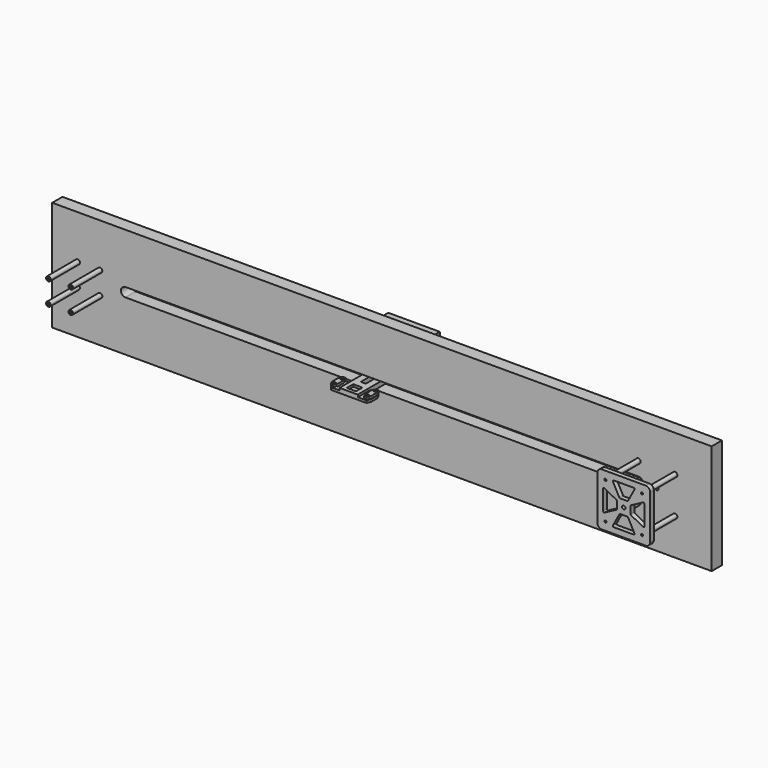
from build123d import *

# Parameters (mm, degrees)
F1_DEPTH       = 6
F2_W           = 8
F2_H           = 7.235
F3_DEPTH       = 6
F6_DEPTH       = 7.62
F8_DEPTH       = 7.62
F9_W           = 8
F9_H           = 3.175
F10_DEPTH      = 7.62
F10_DEPTH_BACK = 13.62
F12_DEPTH      = 7.236
F14_DEPTH      = 19.05
F14_DEPTH_BACK = 3.81
F17_DEPTH      = 7.236
F18_W          = 6.3396086097
F18_H          = 5.2124624596
F18_W_2        = 12.7207827806
F18_H_2        = 4.8503658202
F18_W_3        = 6.3603913903
F19_DEPTH      = 3.175
F19_DEPTH_BACK = 3.175
F20_R          = 1.905
F21_DEPTH      = 6.351
F22_W          = 7.0159770548
F22_H          = 37.1222775429
F23_DEPTH      = 6.351
F26_DEPTH      = 19.05
F27_W          = 15.0859798895
F27_H          = 38.1
F28_DEPTH      = 6.35
F29_TEXT_SIZE  = 21.1979624712
F30_DEPTH      = 3.175
F32_W          = 914.4
F32_H          = 152.4
F32_R          = 1.24968
F32_R_2        = 2.38125
F33_DEPTH      = 17.78
F34_R          = 3.175
F34_R_2        = 1.4605
F35_DEPTH      = 50.8
F36_R          = 1.4605
F36_R_2        = 2.38125
F37_DEPTH      = 6.35


# Not quite as in the source:
# - Text() gives the source's letters only with a copy of the font that has no kerning and outlines rounded to 1/6400 em; it was checked with that copy


with BuildPart() as f1:
    # F0 (on Front) → F1 (new body)
    with BuildSketch(Plane.XZ):
        with BuildLine():
            Line((0.2044851016, 0), (0, 0))
            Line((0, 0), (0, -0.76))
            Line((0, -0.76), (16, -0.76))
            Line((16, -0.76), (16, 0))
            Line((16, 0), (15.7955148984, 0))
            ThreePointArc((15.7955148984, 0), (15.7149199572, 0.0234912831), (15.6595687304, 0.0866072607))
            Line((15.6595687304, 0.0866072607), (15.3859461681, 0.6733927393))
            ThreePointArc((15.3859461681, 0.6733927393), (15.3305949413, 0.7365087169), (15.25, 0.76))
            Line((15.25, 0.76), (14.75, 0.76))
            ThreePointArc((14.75, 0.76), (14.6694050587, 0.7365087169), (14.6140538319, 0.6733927393))
            Line((14.6140538319, 0.6733927393), (14.3404312696, 0.0866072607))
            ThreePointArc((14.3404312696, 0.0866072607), (14.2850800428, 0.0234912831), (14.2044851016, 0))
            Line((14.2044851016, 0), (14, 0))
            Line((14, 0), (13.7955148984, 0))
            ThreePointArc((13.7955148984, 0), (13.7149199572, 0.0234912831), (13.6595687304, 0.0866072607))
            Line((13.6595687304, 0.0866072607), (13.3859461681, 0.6733927393))
            ThreePointArc((13.3859461681, 0.6733927393), (13.3305949413, 0.7365087169), (13.25, 0.76))
            Line((13.25, 0.76), (12.75, 0.76))
            ThreePointArc((12.75, 0.76), (12.6694050587, 0.7365087169), (12.6140538319, 0.6733927393))
            Line((12.6140538319, 0.6733927393), (12.3404312696, 0.0866072607))
            ThreePointArc((12.3404312696, 0.0866072607), (12.2850800428, 0.0234912831), (12.2044851016, 0))
            Line((12.2044851016, 0), (12, 0))
            Line((12, 0), (11.7955148984, 0))
            ThreePointArc((11.7955148984, 0), (11.7149199572, 0.0234912831), (11.6595687304, 0.0866072607))
            Line((11.6595687304, 0.0866072607), (11.3859461681, 0.6733927393))
            ThreePointArc((11.3859461681, 0.6733927393), (11.3305949413, 0.7365087169), (11.25, 0.76))
            Line((11.25, 0.76), (10.75, 0.76))
            ThreePointArc((10.75, 0.76), (10.6694050587, 0.7365087169), (10.6140538319, 0.6733927393))
            Line((10.6140538319, 0.6733927393), (10.3404312696, 0.0866072607))
            ThreePointArc((10.3404312696, 0.0866072607), (10.2850800428, 0.0234912831), (10.2044851016, 0))
            Line((10.2044851016, 0), (10, 0))
            Line((10, 0), (9.7955148984, 0))
            ThreePointArc((9.7955148984, 0), (9.7149199572, 0.0234912831), (9.6595687304, 0.0866072607))
            Line((9.6595687304, 0.0866072607), (9.3859461681, 0.6733927393))
            ThreePointArc((9.3859461681, 0.6733927393), (9.3305949413, 0.7365087169), (9.25, 0.76))
            Line((9.25, 0.76), (8.75, 0.76))
            ThreePointArc((8.75, 0.76), (8.6694050587, 0.7365087169), (8.6140538319, 0.6733927393))
            Line((8.6140538319, 0.6733927393), (8.3404312696, 0.0866072607))
            ThreePointArc((8.3404312696, 0.0866072607), (8.2850800428, 0.0234912831), (8.2044851016, 0))
            Line((8.2044851016, 0), (8, 0))
            Line((8, 0), (7.7955148984, 0))
            ThreePointArc((7.7955148984, 0), (7.7149199572, 0.0234912831), (7.6595687304, 0.0866072607))
            Line((7.6595687304, 0.0866072607), (7.3859461681, 0.6733927393))
            ThreePointArc((7.3859461681, 0.6733927393), (7.3305949413, 0.7365087169), (7.25, 0.76))
            Line((7.25, 0.76), (6.75, 0.76))
            ThreePointArc((6.75, 0.76), (6.6694050587, 0.7365087169), (6.6140538319, 0.6733927393))
            Line((6.6140538319, 0.6733927393), (6.3404312696, 0.0866072607))
            ThreePointArc((6.3404312696, 0.0866072607), (6.2850800428, 0.0234912831), (6.2044851016, 0))
            Line((6.2044851016, 0), (6, 0))
            Line((6, 0), (5.7955148984, 0))
            ThreePointArc((5.7955148984, 0), (5.7149199572, 0.0234912831), (5.6595687304, 0.0866072607))
            Line((5.6595687304, 0.0866072607), (5.3859461681, 0.6733927393))
            ThreePointArc((5.3859461681, 0.6733927393), (5.3305949413, 0.7365087169), (5.25, 0.76))
            Line((5.25, 0.76), (4.75, 0.76))
            ThreePointArc((4.75, 0.76), (4.6694050587, 0.7365087169), (4.6140538319, 0.6733927393))
            Line((4.6140538319, 0.6733927393), (4.3404312696, 0.0866072607))
            ThreePointArc((4.3404312696, 0.0866072607), (4.2850800428, 0.0234912831), (4.2044851016, 0))
            Line((4.2044851016, 0), (4, 0))
            Line((4, 0), (3.7955148984, 0))
            ThreePointArc((3.7955148984, 0), (3.7149199572, 0.0234912831), (3.6595687304, 0.0866072607))
            Line((3.6595687304, 0.0866072607), (3.3859461681, 0.6733927393))
            ThreePointArc((3.3859461681, 0.6733927393), (3.3305949413, 0.7365087169), (3.25, 0.76))
            Line((3.25, 0.76), (2.75, 0.76))
            ThreePointArc((2.75, 0.76), (2.6694050587, 0.7365087169), (2.6140538319, 0.6733927393))
            Line((2.6140538319, 0.6733927393), (2.3404312696, 0.0866072607))
            ThreePointArc((2.3404312696, 0.0866072607), (2.2850800428, 0.0234912831), (2.2044851016, 0))
            Line((2.2044851016, 0), (2, 0))
            Line((2, 0), (1.7955148984, 0))
            ThreePointArc((1.7955148984, 0), (1.7149199572, 0.0234912831), (1.6595687304, 0.0866072607))
            Line((1.6595687304, 0.0866072607), (1.3859461681, 0.6733927393))
            ThreePointArc((1.3859461681, 0.6733927393), (1.3305949413, 0.7365087169), (1.25, 0.76))
            Line((1.25, 0.76), (0.75, 0.76))
            ThreePointArc((0.75, 0.76), (0.6694050587, 0.7365087169), (0.6140538319, 0.6733927393))
            Line((0.6140538319, 0.6733927393), (0.3404312696, 0.0866072607))
            ThreePointArc((0.3404312696, 0.0866072607), (0.2850800428, 0.0234912831), (0.2044851016, 0))
        make_face()
    extrude(amount=F1_DEPTH)


with BuildPart() as f3:
    # F2 (on face) → F3 (new body)
    with BuildSketch(Plane.XZ.offset(6)):
        with Locations((4, -0.3175)):
            Rectangle(F2_W, F2_H)
    extrude(amount=-F3_DEPTH)

    # F4: cut F1
    add(f1.part, mode=Mode.SUBTRACT)

    # F5 (on face) → F6 (join)
    with BuildSketch(Plane(origin=(0, 0, 0), x_dir=(-1, 0, 0), z_dir=(0, 1, 0))):
        with BuildLine():
            Line((0, 0), (0, 3.3))
            Line((0, 3.3), (-8, 3.3))
            Line((-8, 3.3), (-8, 0))
            Line((-8, 0), (-7.7955148984, 0))
            ThreePointArc((-7.7955148984, 0), (-7.7149199572, 0.0234912831), (-7.6595687304, 0.0866072607))
            Line((-7.6595687304, 0.0866072607), (-7.3859461681, 0.6733927393))
            ThreePointArc((-7.3859461681, 0.6733927393), (-7.3305949413, 0.7365087169), (-7.25, 0.76))
            Line((-7.25, 0.76), (-6.75, 0.76))
            ThreePointArc((-6.75, 0.76), (-6.6694050587, 0.7365087169), (-6.6140538319, 0.6733927393))
            Line((-6.6140538319, 0.6733927393), (-6.3404312696, 0.0866072607))
            ThreePointArc((-6.3404312696, 0.0866072607), (-6.2850800428, 0.0234912831), (-6.2044851016, 0))
            Line((-6.2044851016, 0), (-5.7955148984, 0))
            ThreePointArc((-5.7955148984, 0), (-5.7149199572, 0.0234912831), (-5.6595687304, 0.0866072607))
            Line((-5.6595687304, 0.0866072607), (-5.3859461681, 0.6733927393))
            ThreePointArc((-5.3859461681, 0.6733927393), (-5.3305949413, 0.7365087169), (-5.25, 0.76))
            Line((-5.25, 0.76), (-4.75, 0.76))
            ThreePointArc((-4.75, 0.76), (-4.6694050587, 0.7365087169), (-4.6140538319, 0.6733927393))
            Line((-4.6140538319, 0.6733927393), (-4.3404312696, 0.0866072607))
            ThreePointArc((-4.3404312696, 0.0866072607), (-4.2850800428, 0.0234912831), (-4.2044851016, 0))
            Line((-4.2044851016, 0), (-3.7955148984, 0))
            ThreePointArc((-3.7955148984, 0), (-3.7149199572, 0.0234912831), (-3.6595687304, 0.0866072607))
            Line((-3.6595687304, 0.0866072607), (-3.3859461681, 0.6733927393))
            ThreePointArc((-3.3859461681, 0.6733927393), (-3.3305949413, 0.7365087169), (-3.25, 0.76))
            Line((-3.25, 0.76), (-2.75, 0.76))
            ThreePointArc((-2.75, 0.76), (-2.6694050587, 0.7365087169), (-2.6140538319, 0.6733927393))
            Line((-2.6140538319, 0.6733927393), (-2.3404312696, 0.0866072607))
            ThreePointArc((-2.3404312696, 0.0866072607), (-2.2850800428, 0.0234912831), (-2.2044851016, 0))
            Line((-2.2044851016, 0), (-1.7955148984, 0))
            ThreePointArc((-1.7955148984, 0), (-1.7149199572, 0.0234912831), (-1.6595687304, 0.0866072607))
            Line((-1.6595687304, 0.0866072607), (-1.3859461681, 0.6733927393))
            ThreePointArc((-1.3859461681, 0.6733927393), (-1.3305949413, 0.7365087169), (-1.25, 0.76))
            Line((-1.25, 0.76), (-0.75, 0.76))
            ThreePointArc((-0.75, 0.76), (-0.6694050587, 0.7365087169), (-0.6140538319, 0.6733927393))
            Line((-0.6140538319, 0.6733927393), (-0.3404312696, 0.0866072607))
            ThreePointArc((-0.3404312696, 0.0866072607), (-0.2850800428, 0.0234912831), (-0.2044851016, 0))
            Line((-0.2044851016, 0), (0, 0))
        make_face()
    extrude(amount=F6_DEPTH)

    # F7 (on face) → F8 (join)
    with BuildSketch(Plane.XZ.offset(6)):
        with BuildLine():
            Line((8, 0), (8, 3.3))
            Line((8, 3.3), (0, 3.3))
            Line((0, 3.3), (0, 0))
            Line((0, 0), (0.2044851016, 0))
            ThreePointArc((0.2044851016, 0), (0.2850800428, 0.0234912831), (0.3404312696, 0.0866072607))
            Line((0.3404312696, 0.0866072607), (0.6140538319, 0.6733927393))
            ThreePointArc((0.6140538319, 0.6733927393), (0.6694050587, 0.7365087169), (0.75, 0.76))
            Line((0.75, 0.76), (1.25, 0.76))
            ThreePointArc((1.25, 0.76), (1.3305949413, 0.7365087169), (1.3859461681, 0.6733927393))
            Line((1.3859461681, 0.6733927393), (1.6595687304, 0.0866072607))
            ThreePointArc((1.6595687304, 0.0866072607), (1.7149199572, 0.0234912831), (1.7955148984, 0))
            Line((1.7955148984, 0), (2.2044851016, 0))
            ThreePointArc((2.2044851016, 0), (2.2850800428, 0.0234912831), (2.3404312696, 0.0866072607))
            Line((2.3404312696, 0.0866072607), (2.6140538319, 0.6733927393))
            ThreePointArc((2.6140538319, 0.6733927393), (2.6694050587, 0.7365087169), (2.75, 0.76))
            Line((2.75, 0.76), (3.25, 0.76))
            ThreePointArc((3.25, 0.76), (3.3305949413, 0.7365087169), (3.3859461681, 0.6733927393))
            Line((3.3859461681, 0.6733927393), (3.6595687304, 0.0866072607))
            ThreePointArc((3.6595687304, 0.0866072607), (3.7149199572, 0.0234912831), (3.7955148984, 0))
            Line((3.7955148984, 0), (4.2044851016, 0))
            ThreePointArc((4.2044851016, 0), (4.2850800428, 0.0234912831), (4.3404312696, 0.0866072607))
            Line((4.3404312696, 0.0866072607), (4.6140538319, 0.6733927393))
            ThreePointArc((4.6140538319, 0.6733927393), (4.6694050587, 0.7365087169), (4.75, 0.76))
            Line((4.75, 0.76), (5.25, 0.76))
            ThreePointArc((5.25, 0.76), (5.3305949413, 0.7365087169), (5.3859461681, 0.6733927393))
            Line((5.3859461681, 0.6733927393), (5.6595687304, 0.0866072607))
            ThreePointArc((5.6595687304, 0.0866072607), (5.7149199572, 0.0234912831), (5.7955148984, 0))
            Line((5.7955148984, 0), (6.2044851016, 0))
            ThreePointArc((6.2044851016, 0), (6.2850800428, 0.0234912831), (6.3404312696, 0.0866072607))
            Line((6.3404312696, 0.0866072607), (6.6140538319, 0.6733927393))
            ThreePointArc((6.6140538319, 0.6733927393), (6.6694050587, 0.7365087169), (6.75, 0.76))
            Line((6.75, 0.76), (7.25, 0.76))
            ThreePointArc((7.25, 0.76), (7.3305949413, 0.7365087169), (7.3859461681, 0.6733927393))
            Line((7.3859461681, 0.6733927393), (7.6595687304, 0.0866072607))
            ThreePointArc((7.6595687304, 0.0866072607), (7.7149199572, 0.0234912831), (7.7955148984, 0))
            Line((7.7955148984, 0), (8, 0))
        make_face()
    extrude(amount=F8_DEPTH)

    # F9 (on face) → F10 (join, two sides)
    with BuildSketch(Plane(origin=(0, 0, 0), x_dir=(-1, 0, 0), z_dir=(0, 1, 0))) as f10_sk:
        with Locations((-4, -2.3475)):
            Rectangle(F9_W, F9_H)
    extrude(amount=F10_DEPTH)
    extrude(f10_sk.sketch, amount=-F10_DEPTH_BACK)

    # F11 (on face) → F12 (cut, through all)
    with BuildSketch(Plane.XY.offset(3.3)):
        Polygon((8, -13.62), (8, -8.54), (5.5875, -13.62), align=None)
        Polygon((0, -13.62), (2.4125, -13.62), (0, -8.54), align=None)
        Polygon((5.5875, 7.62), (8, 2.54), (8, 7.62), align=None)
        Polygon((0, 7.62), (0, 2.54), (2.4125, 7.62), align=None)
    extrude(amount=-F12_DEPTH, mode=Mode.SUBTRACT)

    # F13 (on face) → F14 (join, two sides)
    with BuildSketch(Plane(origin=(0, 0, 0), x_dir=(0, -1, 0), z_dir=(-1, 0, 0))) as f14_sk:
        Polygon((-7.62, -0.76), (-7.62, -3.935), (-2.54, -3.935), (8.54, -3.935), (13.62, -3.935), (13.62, -0.76), (8.54, -0.76), (-2.54, -0.76), align=None)
    extrude(amount=F14_DEPTH)
    extrude(f14_sk.sketch, amount=-F14_DEPTH_BACK)

    # F15: F3 across face


with BuildPart() as f3_1:
    add(f3.part)
    add(f3.part.mirror(Plane(origin=(-19.05, -3, -2.3475), x_dir=(0, -1, 0), z_dir=(-1, 0, 0))))

    # F16 (on face) → F17 (cut, through all)
    with BuildSketch(Plane.XY.offset(3.3)):
        with BuildLine():
            Line((4.064, 3.35), (2.413, 3.35))
            ThreePointArc((2.413, 3.35), (2.8965667043, 2.1825667043), (4.064, 1.699))
            Line((4.064, 1.699), (4.064, 3.35))
        make_face()
        with BuildLine():
            ThreePointArc((5.715, 3.35), (4.064, 5.001), (2.413, 3.35))
            Line((2.413, 3.35), (4.064, 3.35))
            Line((4.064, 3.35), (4.064, 1.699))
            ThreePointArc((4.064, 1.699), (5.2314332957, 2.1825667043), (5.715, 3.35))
        make_face()
        with BuildLine():
            Line((4.064, -9.35), (4.064, -7.699))
            ThreePointArc((4.064, -7.699), (2.8965667043, -8.1825667043), (2.413, -9.35))
            Line((2.413, -9.35), (4.064, -9.35))
        make_face()
        with BuildLine():
            ThreePointArc((5.715, -9.35), (5.2314332957, -8.1825667043), (4.064, -7.699))
            Line((4.064, -7.699), (4.064, -9.35))
            Line((4.064, -9.35), (2.413, -9.35))
            ThreePointArc((2.413, -9.35), (4.064, -11.001), (5.715, -9.35))
        make_face()
        with BuildLine():
            Line((-42.164, 3.35), (-40.513, 3.35))
            ThreePointArc((-40.513, 3.35), (-43.3314332957, 4.5174332957), (-42.164, 1.699))
            Line((-42.164, 1.699), (-42.164, 3.35))
        make_face()
        with BuildLine():
            ThreePointArc((-42.164, 1.699), (-40.9965667043, 2.1825667043), (-40.513, 3.35))
            Line((-40.513, 3.35), (-42.164, 3.35))
            Line((-42.164, 3.35), (-42.164, 1.699))
        make_face()
        with BuildLine():
            Line((-42.164, -9.35), (-42.164, -7.699))
            ThreePointArc((-42.164, -7.699), (-43.3314332957, -10.5174332957), (-40.513, -9.35))
            Line((-40.513, -9.35), (-42.164, -9.35))
        make_face()
        with BuildLine():
            ThreePointArc((-40.513, -9.35), (-40.9965667043, -8.1825667043), (-42.164, -7.699))
            Line((-42.164, -7.699), (-42.164, -9.35))
            Line((-42.164, -9.35), (-40.513, -9.35))
        make_face()
    extrude(amount=-F17_DEPTH, mode=Mode.SUBTRACT)

    # F18 (on face) → F19 (join, two sides)
    with BuildSketch(Plane.XY.offset(-0.76)) as f19_sk:
        Polygon((-12.6896086097, -8.7696341798), (-6.35, -8.7696341798), (-6.35, 2.4075375404), (-12.6896086097, 2.4075375404), (-12.6896086097, -3), align=None)
        with Locations((-9.5198043048, 5.0137687702)):
            Rectangle(F18_W, F18_H)
        with Locations((-19.05, 5.0137687702)):
            Rectangle(F18_W_2, F18_H)
        with Locations((-28.5801956952, 5.0137687702)):
            Rectangle(F18_W, F18_H)
        Polygon((-31.75, -8.7696341798), (-25.4103913903, -8.7696341798), (-25.4103913903, -3), (-25.4103913903, 2.4075375404), (-31.75, 2.4075375404), align=None)
        with Locations((-28.5801956952, -11.1948170899)):
            Rectangle(F18_W, F18_H_2)
        with Locations((-15.8698043048, -11.1948170899)):
            Rectangle(F18_W_3, F18_H_2)
        with Locations((-22.2301956952, -11.1948170899)):
            Rectangle(F18_W_3, F18_H_2)
        with Locations((-9.5198043048, -11.1948170899)):
            Rectangle(F18_W, F18_H_2)
        with BuildLine():
            Line((-12.6896086097, 7.62), (-6.35, 7.62))
            Line((-6.35, 7.62), (-6.35, 71.12))
            ThreePointArc((-6.35, 71.12), (-19.05, 83.82), (-31.75, 71.12))
            Line((-31.75, 71.12), (-31.75, 7.62))
            Line((-31.75, 7.62), (-25.4103913903, 7.62))
            Line((-25.4103913903, 7.62), (-12.6896086097, 7.62))
        make_face()
    extrude(amount=F19_DEPTH)
    extrude(f19_sk.sketch, amount=-F19_DEPTH_BACK)

    # F20 (on face) → F21 (cut, through all)
    with BuildSketch(Plane.XY.offset(2.415)):
        with BuildLine():
            ThreePointArc((-16.1925, 72.2575375404), (-14.2875, 70.3525375404), (-12.3825, 72.2575375404))
            ThreePointArc((-12.3825, 72.2575375404), (-14.2875, 74.1625375404), (-16.1925, 72.2575375404))
        make_face()
        with Locations((-23.8125, 72.2575375404)):
            Circle(F20_R)
    extrude(amount=-F21_DEPTH, mode=Mode.SUBTRACT)

    # F22 (on face) → F23 (cut, through all)
    with BuildSketch(Plane.XY.offset(2.415)):
        with Locations((-19.022686407, 30.2847372368)):
            Rectangle(F22_W, F22_H)
    extrude(amount=-F23_DEPTH, mode=Mode.SUBTRACT)


with BuildPart() as f26:
    # F25 (on 3pt) → F26 (new body, symmetric)
    with BuildSketch(Plane.XZ.offset(-71.12)):
        Polygon((-19.05, 8.765), (31.75, 8.765), (44.45, 34.165), (-19.05, 34.165), align=None)
        Polygon((-69.85, 8.765), (-19.05, 8.765), (-19.05, 34.165), (-82.55, 34.165), align=None)
    extrude(amount=F26_DEPTH, both=True)

    # F27 (on face) → F28 (join)
    with BuildSketch(Plane.XY.offset(34.165)):
        with Locations((24.2070100553, 71.12)):
            Rectangle(F27_W, F27_H)
        Polygon((16.6640201105, 42.545), (16.6640201105, 52.07), (4.7593467403, 52.07), align=None)
        Polygon((4.7593467403, 52.07), (16.6640201105, 52.07), (16.6640201105, 90.17), (-42.8593467403, 90.17), align=None)
        Polygon((16.6640201105, 42.545), (4.7593467403, 52.07), (-54.7640201105, 52.07), (-54.7640201105, 42.545), align=None)
        Polygon((-54.7640201105, 52.07), (4.7593467403, 52.07), (-42.8593467403, 90.17), (-54.7640201105, 90.17), align=None)
        Polygon((-42.8593467403, 90.17), (16.6640201105, 90.17), (16.6640201105, 99.695), (-54.7640201105, 99.695), align=None)
        with Locations((-62.3070100553, 71.12)):
            Rectangle(F27_W, F27_H)
        Polygon((-54.7640201105, 90.17), (-42.8593467403, 90.17), (-54.7640201105, 99.695), align=None)
    extrude(amount=F28_DEPTH)

    # F29 (on face) → F30 (cut)
    with BuildSketch(Plane.XY.offset(40.515)):
        with Locations((-30.2830450237, 47.0722429454)):
            Text('X', F29_TEXT_SIZE, font='Open Sans', text_align=(TextAlign.LEFT, TextAlign.BOTTOM))
    extrude(amount=-F30_DEPTH, mode=Mode.SUBTRACT)


with BuildPart() as f33:
    # F32 (on offset) → F33 (new body)
    with BuildSketch(Plane.XZ.offset(-20.32)):
        Rectangle(F32_W, F32_H)
        with Locations((-421.90035, -15.50035)):
            Circle(F32_R, mode=Mode.SUBTRACT)
        with Locations((-390.89965, -15.50035)):
            Circle(F32_R, mode=Mode.SUBTRACT)
        with Locations((355.6, -25.4)):
            Circle(F32_R, mode=Mode.SUBTRACT)
        with Locations((406.4, -25.4)):
            Circle(F32_R, mode=Mode.SUBTRACT)
        with Locations((-421.90035, 15.50035)):
            Circle(F32_R, mode=Mode.SUBTRACT)
        with Locations((-390.89965, 15.50035)):
            Circle(F32_R, mode=Mode.SUBTRACT)
        with BuildLine():
            Line((-355.6, 6.35), (355.6, 6.35))
            ThreePointArc((355.6, 6.35), (361.95, 0), (355.6, -6.35))
            Line((355.6, -6.35), (-355.6, -6.35))
            ThreePointArc((-355.6, -6.35), (-361.95, 0), (-355.6, 6.35))
        make_face(mode=Mode.SUBTRACT)
        with Locations((381, 0)):
            Circle(F32_R_2, mode=Mode.SUBTRACT)
        with Locations((355.6, 25.4)):
            Circle(F32_R, mode=Mode.SUBTRACT)
        with Locations((406.4, 25.4)):
            Circle(F32_R, mode=Mode.SUBTRACT)
    extrude(amount=-F33_DEPTH)


with BuildPart() as f35:
    # F34 (on face) → F35 (new body)
    with BuildSketch(Plane.XZ.offset(-20.32)):
        with Locations((-421.90035, 15.50035)):
            Circle(F34_R)
        with Locations((-421.90035, 15.50035)):
            Circle(F34_R_2, mode=Mode.SUBTRACT)
    extrude(amount=F35_DEPTH)


with BuildPart() as f35b:
    # F34 (on face) → F35, piece 2 (new body)
    with BuildSketch(Plane.XZ.offset(-20.32)):
        with Locations((-390.89965, 15.50035)):
            Circle(F34_R)
        with Locations((-390.89965, 15.50035)):
            Circle(F34_R_2, mode=Mode.SUBTRACT)
    extrude(amount=F35_DEPTH)


with BuildPart() as f35c:
    # F34 (on face) → F35, piece 3 (new body)
    with BuildSketch(Plane.XZ.offset(-20.32)):
        with Locations((-390.89965, -15.50035)):
            Circle(F34_R)
        with Locations((-390.89965, -15.50035)):
            Circle(F34_R_2, mode=Mode.SUBTRACT)
    extrude(amount=F35_DEPTH)


with BuildPart() as f35d:
    # F34 (on face) → F35, piece 4 (new body)
    with BuildSketch(Plane.XZ.offset(-20.32)):
        with Locations((-421.90035, -15.50035)):
            Circle(F34_R)
        with Locations((-421.90035, -15.50035)):
            Circle(F34_R_2, mode=Mode.SUBTRACT)
    extrude(amount=F35_DEPTH)


with BuildPart() as f35e:
    # F34 (on face) → F35, piece 5 (new body)
    with BuildSketch(Plane.XZ.offset(-20.32)):
        with Locations((406.4, 25.4)):
            Circle(F34_R)
        with Locations((406.4, 25.4)):
            Circle(F34_R_2, mode=Mode.SUBTRACT)
    extrude(amount=F35_DEPTH)


with BuildPart() as f35f:
    # F34 (on face) → F35, piece 6 (new body)
    with BuildSketch(Plane.XZ.offset(-20.32)):
        with Locations((355.6, 25.4)):
            Circle(F34_R)
        with Locations((355.6, 25.4)):
            Circle(F34_R_2, mode=Mode.SUBTRACT)
    extrude(amount=F35_DEPTH)


with BuildPart() as f35g:
    # F34 (on face) → F35, piece 7 (new body)
    with BuildSketch(Plane.XZ.offset(-20.32)):
        with Locations((355.6, -25.4)):
            Circle(F34_R)
        with Locations((355.6, -25.4)):
            Circle(F34_R_2, mode=Mode.SUBTRACT)
    extrude(amount=F35_DEPTH)


with BuildPart() as f35h:
    # F34 (on face) → F35, piece 8 (new body)
    with BuildSketch(Plane.XZ.offset(-20.32)):
        with Locations((406.4, -25.4)):
            Circle(F34_R)
        with Locations((406.4, -25.4)):
            Circle(F34_R_2, mode=Mode.SUBTRACT)
    extrude(amount=F35_DEPTH)


with BuildPart() as f37:
    # F36 (on face) → F37 (new body)
    with BuildSketch(Plane.XZ.offset(30.48)):
        with BuildLine():
            ThreePointArc((417.6395, 30.2895), (415.7796280605, 34.7796280605), (411.2895, 36.6395))
            Line((411.2895, 36.6395), (350.7105, 36.6395))
            ThreePointArc((350.7105, 36.6395), (346.2203719395, 34.7796280605), (344.3605, 30.2895))
            Line((344.3605, 30.2895), (344.3605, -30.2895))
            ThreePointArc((344.3605, -30.2895), (346.2203719395, -34.7796280605), (350.7105, -36.6395))
            Line((350.7105, -36.6395), (411.2895, -36.6395))
            ThreePointArc((411.2895, -36.6395), (415.7796280605, -34.7796280605), (417.6395, -30.2895))
            Line((417.6395, -30.2895), (417.6395, 30.2895))
        make_face()
        with Locations((355.6, -25.4)):
            Circle(F36_R, mode=Mode.SUBTRACT)
        with BuildLine():
            Line((394.7583333333, -28.575), (367.2416666667, -28.575))
            ThreePointArc((367.2416666667, -28.575), (366.152650651, -27.9584096094), (366.1210784314, -26.7073529412))
            Line((366.1210784314, -26.7073529412), (374.9264117647, -10.1973529412))
            ThreePointArc((374.9264117647, -10.1973529412), (375.3935903906, -9.7059839843), (376.047, -9.525))
            Line((376.047, -9.525), (385.953, -9.525))
            ThreePointArc((385.953, -9.525), (386.6064096094, -9.7059839843), (387.0735882353, -10.1973529412))
            Line((387.0735882353, -10.1973529412), (395.8789215686, -26.7073529412))
            ThreePointArc((395.8789215686, -26.7073529412), (395.847349349, -27.9584096094), (394.7583333333, -28.575))
        make_face(mode=Mode.SUBTRACT)
        with Locations((406.4, -25.4)):
            Circle(F36_R, mode=Mode.SUBTRACT)
        with BuildLine():
            Line((352.425, -13.7583333333), (352.425, 13.7583333333))
            ThreePointArc((352.425, 13.7583333333), (353.0415903906, 14.847349349), (354.2926470588, 14.8789215686))
            Line((354.2926470588, 14.8789215686), (370.8026470588, 6.0735882353))
            ThreePointArc((370.8026470588, 6.0735882353), (371.2940160156, 5.6064096094), (371.475, 4.953))
            Line((371.475, 4.953), (371.475, -4.953))
            ThreePointArc((371.475, -4.953), (371.2940160156, -5.6064096094), (370.8026470588, -6.0735882353))
            Line((370.8026470588, -6.0735882353), (354.2926470588, -14.8789215686))
            ThreePointArc((354.2926470588, -14.8789215686), (353.0415903906, -14.847349349), (352.425, -13.7583333333))
        make_face(mode=Mode.SUBTRACT)
        with Locations((381, 0)):
            Circle(F36_R_2, mode=Mode.SUBTRACT)
        with Locations((355.6, 25.4)):
            Circle(F36_R, mode=Mode.SUBTRACT)
        with BuildLine():
            ThreePointArc((366.1210784314, 26.7073529412), (366.152650651, 27.9584096094), (367.2416666667, 28.575))
            Line((367.2416666667, 28.575), (394.7583333333, 28.575))
            ThreePointArc((394.7583333333, 28.575), (395.847349349, 27.9584096094), (395.8789215686, 26.7073529412))
            Line((395.8789215686, 26.7073529412), (387.0735882353, 10.1973529412))
            ThreePointArc((387.0735882353, 10.1973529412), (386.6064096094, 9.7059839843), (385.953, 9.525))
            Line((385.953, 9.525), (376.047, 9.525))
            ThreePointArc((376.047, 9.525), (375.3935903906, 9.7059839843), (374.9264117647, 10.1973529412))
            Line((374.9264117647, 10.1973529412), (366.1210784314, 26.7073529412))
        make_face(mode=Mode.SUBTRACT)
        with BuildLine():
            Line((391.1973529412, 6.0735882353), (407.7073529412, 14.8789215686))
            ThreePointArc((407.7073529412, 14.8789215686), (408.9584096094, 14.847349349), (409.575, 13.7583333333))
            Line((409.575, 13.7583333333), (409.575, -13.7583333333))
            ThreePointArc((409.575, -13.7583333333), (408.9584096094, -14.847349349), (407.7073529412, -14.8789215686))
            Line((407.7073529412, -14.8789215686), (391.1973529412, -6.0735882353))
            ThreePointArc((391.1973529412, -6.0735882353), (390.7059839843, -5.6064096094), (390.525, -4.953))
            Line((390.525, -4.953), (390.525, 4.953))
            ThreePointArc((390.525, 4.953), (390.7059839843, 5.6064096094), (391.1973529412, 6.0735882353))
        make_face(mode=Mode.SUBTRACT)
        with Locations((406.4, 25.4)):
            Circle(F36_R, mode=Mode.SUBTRACT)
    extrude(amount=F37_DEPTH)


solid = Compound([f3_1.part, f26.part, f33.part, f35.part, f35b.part, f35c.part, f35d.part, f35e.part, f35f.part, f35g.part, f35h.part, f37.part])
